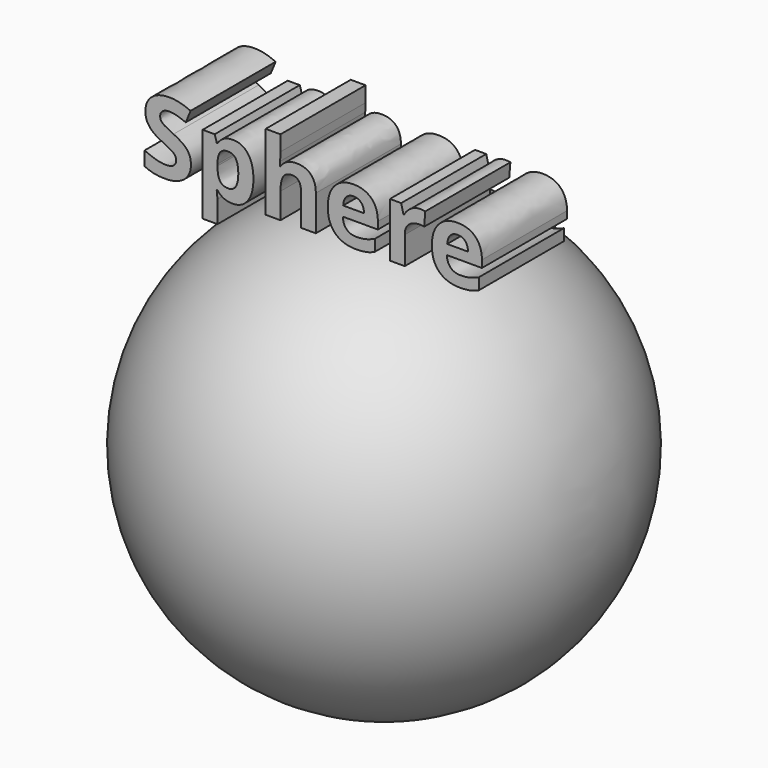
from build123d import *

# Parameters (mm, degrees)
F2_TEXT_SIZE = 23.7835105509
F3_DEPTH     = 25.4


# Not quite as in the source:
# - Text() gives the source's letters only with a copy of the font that has no kerning and outlines rounded to 1/6400 em; it was checked with that copy


with BuildPart() as f1:
    # F0 (on Front) → F1 (revolve)
    with BuildSketch(Plane.XZ):
        with BuildLine():
            ThreePointArc((0, -51.6745696968), (36.5394386475, -36.5394386475), (51.6745696968, 0))
            ThreePointArc((51.6745696968, 0), (36.5394386475, 36.5394386475), (0, 51.6745696968))
            Line((0, 51.6745696968), (0, -51.6745696968))
        make_face()
    revolve(axis=Axis((0, 0, 0), (0, 0, -1)))


with BuildPart() as f3:
    # F2 (on Front) → F3 (new body)
    with BuildSketch(Plane.XZ):
        with Locations((-37.9492528737, 56.1335794628)):
            Text('Sphere', F2_TEXT_SIZE, font='Open Sans', font_style=FontStyle.BOLD, text_align=(TextAlign.LEFT, TextAlign.BOTTOM))
    extrude(amount=F3_DEPTH)


solid = Compound([f1.part, f3.part])
